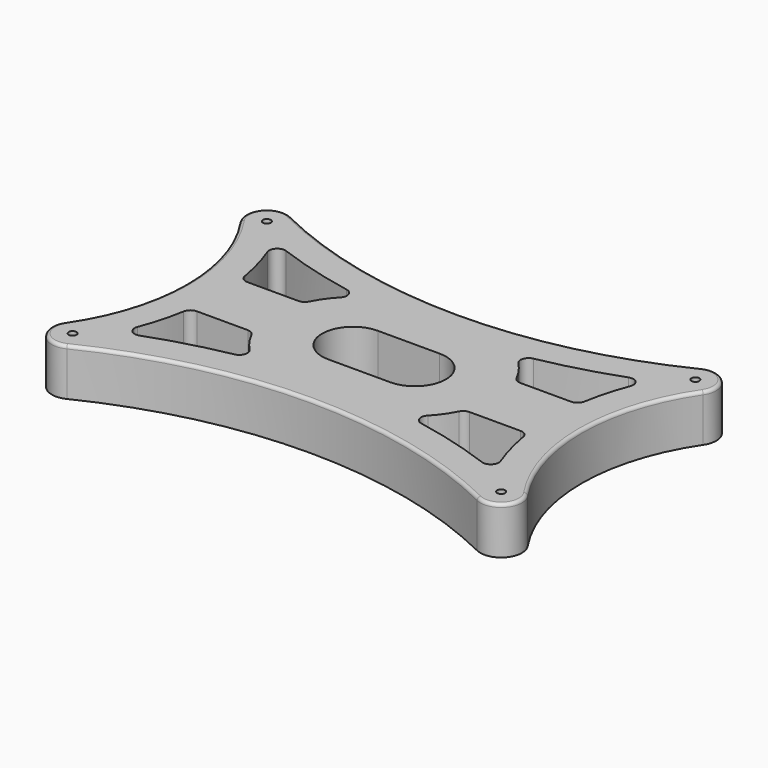
from build123d import *

# Parameters (mm, degrees)
F0_R     = 1.5875
F1_DEPTH = 19.05
F0_R_2   = 3.175
F2_DEPTH = 6.35
F3_R     = 1.27


with BuildPart() as f1:
    # F0 (on Top) → F1 (new body)
    with BuildSketch(Plane.XY):
        with BuildLine():
            ThreePointArc((82.8215071839, 56.5294814298), (0, 37.38), (-82.8215071839, 56.5294814298))
            ThreePointArc((-82.8215071839, 56.5294814298), (-92.8246316261, 54.4975844509), (-93.4439756283, 44.3089870526))
            ThreePointArc((-93.4439756283, 44.3089870526), (-79.88, 0), (-93.4439756283, -44.3089870526))
            ThreePointArc((-93.4439756283, -44.3089870526), (-92.8246316261, -54.4975844509), (-82.8215071839, -56.5294814298))
            ThreePointArc((-82.8215071839, -56.5294814298), (0, -37.38), (82.8215071839, -56.5294814298))
            ThreePointArc((82.8215071839, -56.5294814298), (92.8246316261, -54.4975844509), (93.4439756283, -44.3089870526))
            ThreePointArc((93.4439756283, -44.3089870526), (79.88, 0), (93.4439756283, 44.3089870526))
            ThreePointArc((93.4439756283, 44.3089870526), (92.8246316261, 54.4975844509), (82.8215071839, 56.5294814298))
        make_face()
        with Locations((-86.5, -49)):
            Circle(F0_R, mode=Mode.SUBTRACT)
        with BuildLine():
            ThreePointArc((-44.7490329893, -12.754), (-43.0382407412, -13.2414304642), (-41.8412453259, -14.557333405))
            ThreePointArc((-41.8412453259, -14.557333405), (-39.2272080278, -18.9335940639), (-35.965811948, -22.8512647956))
            ThreePointArc((-35.965811948, -22.8512647956), (-35.1953196756, -26.0911928639), (-37.6837042763, -28.304501317))
            ThreePointArc((-37.6837042763, -28.304501317), (-53.5961461859, -32.0117479156), (-69.1555424288, -36.9971940769))
            ThreePointArc((-69.1555424288, -36.9971940769), (-72.5826288572, -36.2271539786), (-73.3024493232, -32.7891688656))
            ThreePointArc((-73.3024493232, -32.7891688656), (-70.5039949655, -24.2377869494), (-68.556245082, -15.4534970032))
            ThreePointArc((-68.556245082, -15.4534970032), (-67.4497325668, -13.5190259244), (-65.356580963, -12.754))
            Line((-65.356580963, -12.754), (-44.7490329893, -12.754))
        make_face(mode=Mode.SUBTRACT)
        with Locations((86.5, -49)):
            Circle(F0_R, mode=Mode.SUBTRACT)
        with BuildLine():
            ThreePointArc((-12.5, -12.5), (-25, 0), (-12.5, 12.5))
            Line((-12.5, 12.5), (12.5, 12.5))
            ThreePointArc((12.5, 12.5), (25, 0), (12.5, -12.5))
            Line((12.5, -12.5), (-12.5, -12.5))
        make_face(mode=Mode.SUBTRACT)
        with BuildLine():
            ThreePointArc((65.356580963, -12.754), (67.4497325668, -13.5190259244), (68.556245082, -15.4534970032))
            ThreePointArc((68.556245082, -15.4534970032), (70.5039949655, -24.2377869494), (73.3024493232, -32.7891688656))
            ThreePointArc((73.3024493232, -32.7891688656), (72.5826288572, -36.2271539786), (69.1555424288, -36.9971940769))
            ThreePointArc((69.1555424288, -36.9971940769), (53.5961461859, -32.0117479156), (37.6837042763, -28.304501317))
            ThreePointArc((37.6837042763, -28.304501317), (35.1953196756, -26.0911928639), (35.965811948, -22.8512647956))
            ThreePointArc((35.965811948, -22.8512647956), (39.2272080278, -18.9335940639), (41.8412453259, -14.557333405))
            ThreePointArc((41.8412453259, -14.557333405), (43.0382407412, -13.2414304642), (44.7490329893, -12.754))
            Line((44.7490329893, -12.754), (65.356580963, -12.754))
        make_face(mode=Mode.SUBTRACT)
        with BuildLine():
            ThreePointArc((-73.3024493232, 32.7891688656), (-72.5826288572, 36.2271539786), (-69.1555424288, 36.9971940769))
            ThreePointArc((-69.1555424288, 36.9971940769), (-53.5961461859, 32.0117479156), (-37.6837042763, 28.304501317))
            ThreePointArc((-37.6837042763, 28.304501317), (-35.1953196756, 26.0911928639), (-35.965811948, 22.8512647956))
            ThreePointArc((-35.965811948, 22.8512647956), (-39.2272080278, 18.9335940639), (-41.8412453259, 14.557333405))
            ThreePointArc((-41.8412453259, 14.557333405), (-43.0382407412, 13.2414304642), (-44.7490329893, 12.754))
            Line((-44.7490329893, 12.754), (-65.356580963, 12.754))
            ThreePointArc((-65.356580963, 12.754), (-67.4497325668, 13.5190259244), (-68.556245082, 15.4534970032))
            ThreePointArc((-68.556245082, 15.4534970032), (-70.5039949655, 24.2377869494), (-73.3024493232, 32.7891688656))
        make_face(mode=Mode.SUBTRACT)
        with Locations((-86.5, 49)):
            Circle(F0_R, mode=Mode.SUBTRACT)
        with BuildLine():
            ThreePointArc((35.965811948, 22.8512647956), (35.1953196756, 26.0911928639), (37.6837042763, 28.304501317))
            ThreePointArc((37.6837042763, 28.304501317), (53.5961461859, 32.0117479156), (69.1555424288, 36.9971940769))
            ThreePointArc((69.1555424288, 36.9971940769), (72.5826288572, 36.2271539786), (73.3024493232, 32.7891688656))
            ThreePointArc((73.3024493232, 32.7891688656), (70.5039949655, 24.2377869494), (68.556245082, 15.4534970032))
            ThreePointArc((68.556245082, 15.4534970032), (67.4497325668, 13.5190259244), (65.356580963, 12.754))
            Line((65.356580963, 12.754), (44.7490329893, 12.754))
            ThreePointArc((44.7490329893, 12.754), (43.0382407412, 13.2414304642), (41.8412453259, 14.557333405))
            ThreePointArc((41.8412453259, 14.557333405), (39.2272080278, 18.9335940639), (35.965811948, 22.8512647956))
        make_face(mode=Mode.SUBTRACT)
        with Locations((86.5, 49)):
            Circle(F0_R, mode=Mode.SUBTRACT)
    extrude(amount=F1_DEPTH)

    # F0 (on Top) → F2 (cut)
    with BuildSketch(Plane.XY):
        with BuildLine():
            Line((12.5, 12.5), (-12.5, 12.5))
            ThreePointArc((-12.5, 12.5), (-25, 0), (-12.5, -12.5))
            Line((-12.5, -12.5), (12.5, -12.5))
            ThreePointArc((12.5, -12.5), (25, 0), (12.5, 12.5))
        make_face()
        with Locations((-12.5, 0)):
            Circle(F0_R_2, mode=Mode.SUBTRACT)
        with Locations((12.5, 0)):
            Circle(F0_R_2, mode=Mode.SUBTRACT)
    extrude(amount=F2_DEPTH, mode=Mode.SUBTRACT)

    # F3
    f3_edges = [f1.edges().sort_by_distance(p)[0] for p in [
        (-79.88, 0, 19.05),
        (-92.824632, -54.497584, 19.05),
        (0, -37.38, 19.05),
        (92.824632, -54.497584, 19.05),
        (79.88, 0, 19.05),
        (92.824632, 54.497584, 19.05),
        (0, 37.38, 19.05),
        (-92.824632, 54.497584, 19.05),
    ]]
    fillet(f3_edges, radius=F3_R)


solid = f1.part
